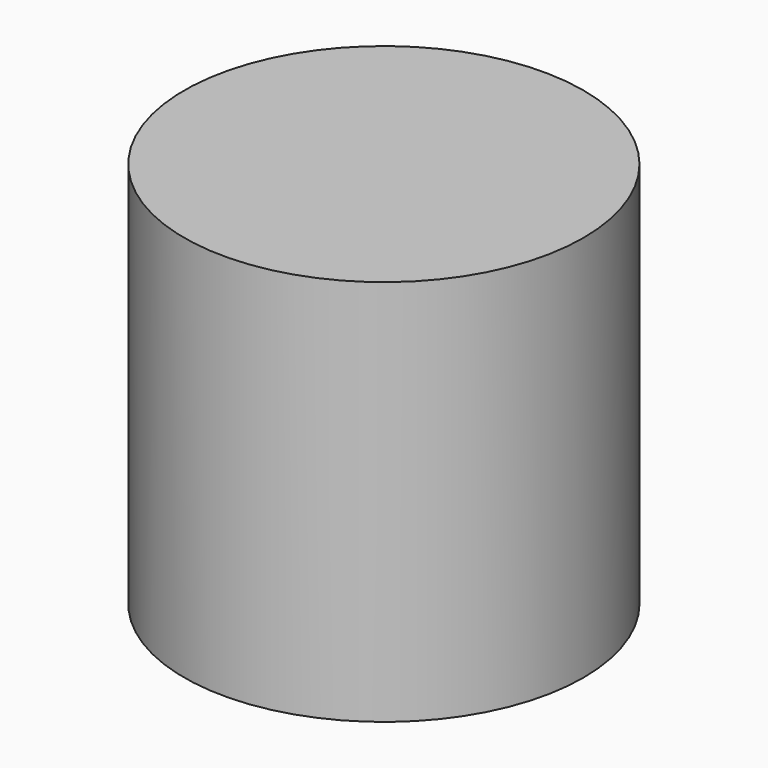
from build123d import *

# Parameters (mm, degrees)
F0_R     = 56.7089177441
F1_DEPTH = 109.982


# Not quite as in the source:
# - the program builds the solid bodies; features that only make, move or delete a surface that nothing else refers to are left out


with BuildPart() as f1:
    # F0 (on Top) → F1 (new body)
    with BuildSketch(Plane.XY):
        Circle(F0_R)
    extrude(amount=F1_DEPTH)


solid = f1.part
